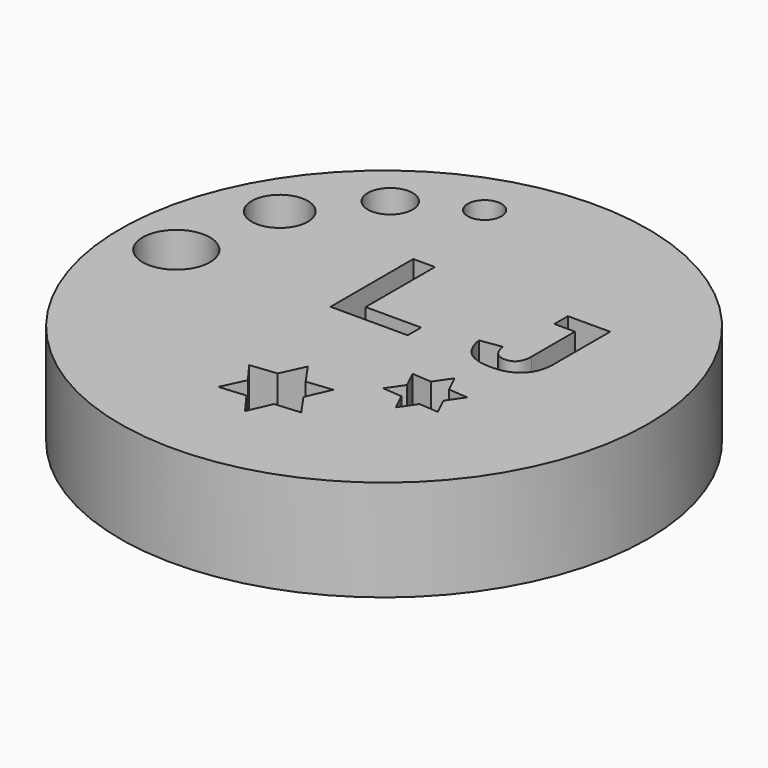
from build123d import *

# Parameters (mm, degrees)
F0_R         = 23.5
F1_DEPTH     = 9
F2_R         = 3
F2_R_2       = 2.5
F2_R_3       = 2
F2_R_4       = 1.5
F2_TEXT_SIZE = 13.3832273051
F3_DEPTH     = 9.001


# Not quite as in the source:
# - Text() gives the source's letters only with a copy of the font that has no kerning and outlines rounded to 1/6400 em; it was checked with that copy


with BuildPart() as f1:
    # F0 (on Top) → F1 (new body)
    with BuildSketch(Plane.XY):
        Circle(F0_R)
    extrude(amount=F1_DEPTH)

    # F2 (on face) → F3 (cut, through all)
    with BuildSketch(Plane.XY.offset(9)):
        with Locations((-18.5, 0)):
            Circle(F2_R)
        with Locations((-16.5, 9.0138781887)):
            Circle(F2_R_2)
        with Locations((-11.4498743711, 15)):
            Circle(F2_R_3)
        with Locations((-5.5, 18.0623918682)):
            Circle(F2_R_4)
        Polygon((1.3161660792, -13.8914508377), (3.5853407901, -13.6971127853), (2.2461797302, -11.7771145133), (3.1886948674, -9.6343567283), (0.9247812535, -9.8825830278), (-0.3781077923, -8.0145891087), (-1.3712945412, -10.1343357424), (-3.6982347857, -10.3894725826), (-2.3513076975, -12.2259661345), (-3.3175933626, -14.2882981059), (-0.9852455539, -14.0885497444), (0.3991795535, -15.9761706891), align=None)
        Polygon((9.2130344691, -7.5693346103), (10.939940208, -7.7027383918), (10.1920184023, -6.1404922612), (11.1710023356, -4.7116499121), (9.4440965966, -4.5782461306), (8.6961747909, -3.016), (7.7171908577, -4.4448423491), (5.9902851188, -4.3114385676), (6.7382069245, -5.8736846982), (5.7592229913, -7.3025270472), (7.4861287302, -7.4359308288), (8.2340505359, -8.9981769593), align=None)
        with Locations((-5.662, 0)):
            Text('L J', F2_TEXT_SIZE, font='Arimo', font_style=FontStyle.BOLD, text_align=(TextAlign.LEFT, TextAlign.BOTTOM))
    extrude(amount=-F3_DEPTH, mode=Mode.SUBTRACT)


solid = f1.part
